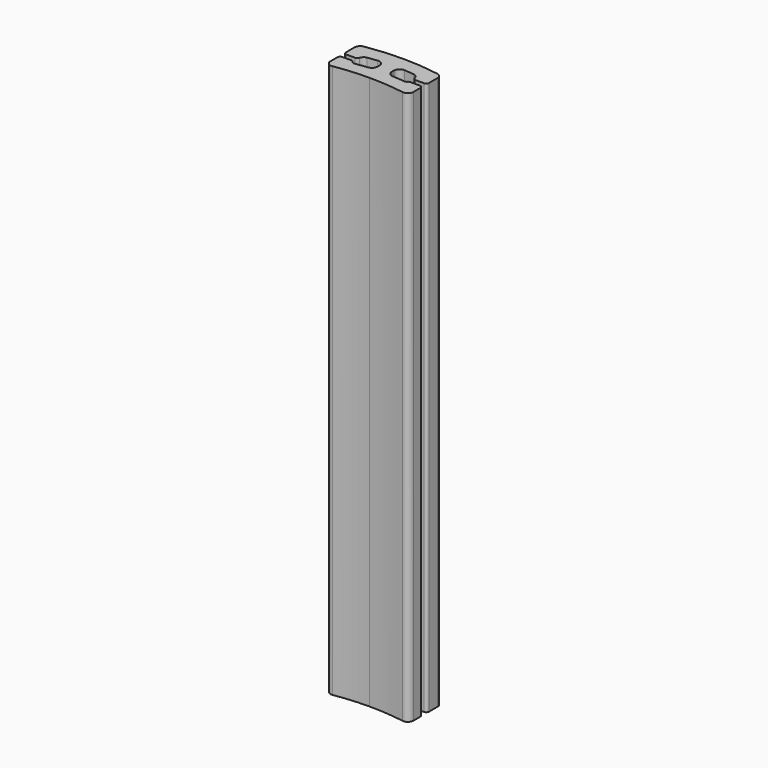
from build123d import *

# Parameters (mm, degrees)
F1_DEPTH    = 254
F2_R        = 2.54
F3_R        = 1.27
F4_T1_DEPTH = 254
F5_R        = 1.27
F6_R        = 1.27
F7_R        = 1.27


# Not quite as in the source:
# - a fillet or chamfer that OpenCascade refuses, or shapes differently, is made with other operations: its cross-section is extruded or revolved along the edge and cut away or added


with BuildPart() as f1:
    # F0 (on Top) → F1 (new body)
    with BuildSketch(Plane.XY):
        with BuildLine():
            ThreePointArc((0, -7.7230836489), (9.5675153846, -8.1745658676), (19.05, -9.525))
            Line((19.05, -9.525), (19.05, -1.190625))
            Line((19.05, -1.190625), (12.7, -1.190625))
            Line((12.7, -1.190625), (12.7, -2.1699586974))
            Line((12.7, -2.1699586974), (3.2042846004, -1.4236249591))
            Line((3.2042846004, -1.4236249591), (3.2042846004, 1.7513750409))
            Line((3.2042846004, 1.7513750409), (3.2042846004, 4.9263750409))
            Line((3.2042846004, 4.9263750409), (12.7, 4.1800413026))
            Line((12.7, 4.1800413026), (12.7, 1.190625))
            Line((12.7, 1.190625), (19.05, 1.190625))
            Line((19.05, 1.190625), (19.05, 9.525))
            ThreePointArc((19.05, 9.525), (0, 11.3269163511), (-19.05, 9.525))
            Line((-19.05, 9.525), (-19.05, 1.190625))
            Line((-19.05, 1.190625), (-12.7, 1.190625))
            Line((-12.7, 1.190625), (-12.7, 3.6498726836))
            Line((-12.7, 3.6498726836), (-3.2606808159, 4.9245798427))
            Line((-3.2606808159, 4.9245798427), (-3.2606808159, 1.7495798427))
            Line((-3.2606808159, 1.7495798427), (-3.2606808159, -1.4254201573))
            Line((-3.2606808159, -1.4254201573), (-12.7, -2.7001273164))
            Line((-12.7, -2.7001273164), (-12.7, -1.190625))
            Line((-12.7, -1.190625), (-19.05, -1.190625))
            Line((-19.05, -1.190625), (-19.05, -9.525))
            ThreePointArc((-19.05, -9.525), (-9.5675153846, -8.1745658676), (0, -7.7230836489))
        make_face()
    extrude(amount=F1_DEPTH)

    # F2
    f2_edges = [f1.edges().sort_by_distance(p)[0] for p in [
        (19.05, -9.525, 127),
        (19.05, 9.525, 127),
        (-19.05, -9.525, 127),
        (-19.05, 9.525, 127),
        (-12.7, 3.649873, 127),
        (3.204285, 4.926375, 127),
        (3.204285, -1.423625, 127),
        (12.7, 4.180041, 127),
        (-3.260681, 4.92458, 127),
        (-3.260681, -1.42542, 127),
    ]]
    fillet(f2_edges, radius=F2_R)

    # F3
    f3_edges = [f1.edges().sort_by_distance(p)[0] for p in [
        (19.05, -1.190625, 127),
        (19.05, 1.190625, 127),
        (-19.05, -1.190625, 127),
        (-19.05, 1.190625, 127),
    ]]
    fillet(f3_edges, radius=F3_R)

    # F4: fillet of radius 1.27 on 1 edges, made by hand

    # F4_s2 → F4_t1 (join)
    with BuildSketch(Plane.XY):
        with BuildLine():
            ThreePointArc((12.7, -1.190625), (12.1981114255, -1.8561294958), (11.3917205019, -2.0671319921))
            Line((11.3917205019, -2.0671319921), (12.7, -2.1699586974))
            Line((12.7, -2.1699586974), (12.7, -1.190625))
        make_face()
    extrude(amount=F4_T1_DEPTH)

    # F5
    f5_edges = [f1.edges().sort_by_distance(p)[0] for p in [
        (-12.7, -2.700127, 127),
    ]]
    fillet(f5_edges, radius=F5_R)

    # F6
    f6_edges = [f1.edges().sort_by_distance(p)[0] for p in [
        (-12.7, 1.190625, 127),
        (-12.7, -1.190625, 127),
        (12.7, 1.190625, 127),
    ]]
    fillet(f6_edges, radius=F6_R)

    # F7
    f7_edges = [f1.edges().sort_by_distance(p)[0] for p in [
        (12.7, -1.190625, 127),
    ]]
    fillet(f7_edges, radius=F7_R)


solid = f1.part
